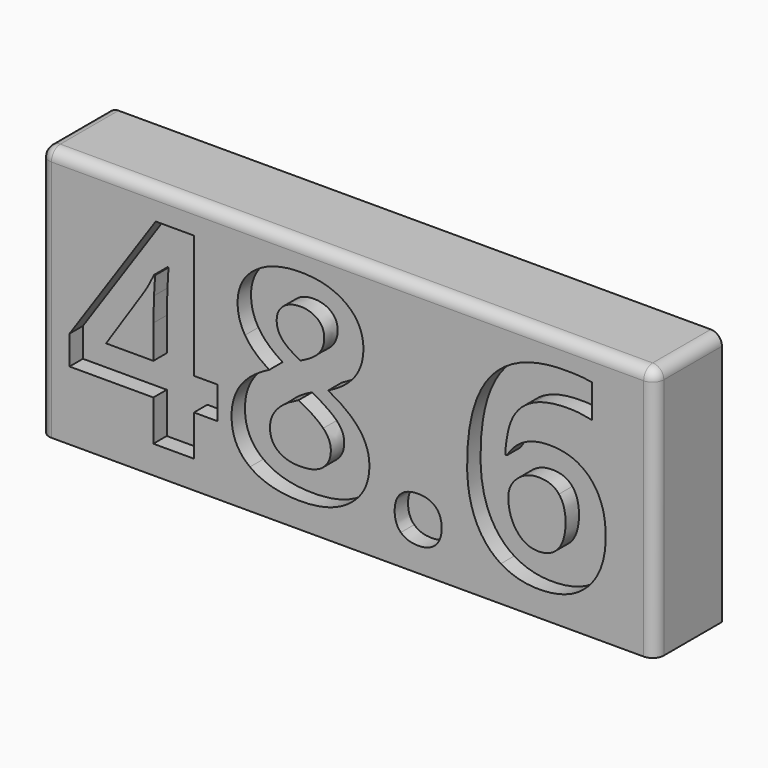
from build123d import *

# Parameters (mm, degrees)
F0_W         = 110
F0_H         = 45.4570637119
F1_DEPTH     = 15
F0_TEXT_SIZE = 49.2459218221
F2_DEPTH     = 12
F3_R         = 2


# Not quite as in the source:
# - Text() gives the source's letters only with a copy of the font that has no kerning and outlines rounded to 1/6400 em; it was checked with that copy


with BuildPart() as f1:
    # F0 (on Front) → F1 (new body)
    with BuildSketch(Plane.XZ):
        with Locations((0.6027820706, 5.2631582404)):
            Rectangle(F0_W, F0_H)
        Polygon((-22.6608187135, 0.5924903425), (-22.6608187135, -5.178516121), (-26.89289012, -5.178516121), (-26.89289012, -12.4653736156), (-34.1566635888, -12.4653736156), (-34.1566635888, -5.178516121), (-49.161280394, -5.178516121), (-49.161280394, -0.0076943297), (-33.7411511234, 22.6915977602), (-26.89289012, 22.6915977602), (-26.89289012, 0.5924903425), align=None, mode=Mode.SUBTRACT)
        with BuildLine():
            add(Edge.make_bspline(
                [(-15.9510618652, 20.8140969907), (-12.8270236996, 23.145583602), (-7.8024007387, 23.145583602)],
                knots=[0, 0, 0, 1, 1, 1], degree=2))
            add(Edge.make_bspline(
                [(-7.8024007387, 23.145583602), (-2.7469990766, 23.145583602), (0.3424130502, 20.8487230295)],
                knots=[0, 0, 0, 1, 1, 1], degree=2))
            add(Edge.make_bspline(
                [(0.3424130502, 20.8487230295), (3.431825177, 18.551862457), (3.431825177, 14.658356763)],
                knots=[0, 0, 0, 1, 1, 1], degree=2))
            add(Edge.make_bspline(
                [(3.431825177, 14.658356763), (3.431825177, 11.9652204133), (1.9390581717, 9.860726723)],
                knots=[0, 0, 0, 1, 1, 1], degree=2))
            add(Edge.make_bspline(
                [(1.9390581717, 9.860726723), (0.4462911665, 7.7562330326), (-2.8701138812, 6.1018778464)],
                knots=[0, 0, 0, 1, 1, 1], degree=2))
            add(Edge.make_bspline(
                [(-2.8701138812, 6.1018778464), (1.0695598646, 3.9858421431), (2.7893197907, 1.6889815706)],
                knots=[0, 0, 0, 1, 1, 1], degree=2))
            add(Edge.make_bspline(
                [(2.7893197907, 1.6889815706), (4.5090797168, -0.6078790019), (4.5090797168, -3.3548780785)],
                knots=[0, 0, 0, 1, 1, 1], degree=2))
            add(Edge.make_bspline(
                [(4.5090797168, -3.3548780785), (4.5090797168, -7.6792855885), (1.1195752539, -10.3147118735)],
                knots=[0, 0, 0, 1, 1, 1], degree=2))
            add(Edge.make_bspline(
                [(1.1195752539, -10.3147118735), (-2.269929209, -12.9501381585), (-7.8024007387, -12.9501381585)],
                knots=[0, 0, 0, 1, 1, 1], degree=2))
            add(Edge.make_bspline(
                [(-7.8024007387, -12.9501381585), (-13.5734072022, -12.9501381585), (-16.8667282241, -10.4955367427)],
                knots=[0, 0, 0, 1, 1, 1], degree=2))
            add(Edge.make_bspline(
                [(-16.8667282241, -10.4955367427), (-20.1600492459, -8.0409353269), (-20.1600492459, -3.5472449606)],
                knots=[0, 0, 0, 1, 1, 1], degree=2))
            add(Edge.make_bspline(
                [(-20.1600492459, -3.5472449606), (-20.1600492459, -0.5386269243), (-18.5595567867, 1.792859687)],
                knots=[0, 0, 0, 1, 1, 1], degree=2))
            add(Edge.make_bspline(
                [(-18.5595567867, 1.792859687), (-16.9590643275, 4.1243462982), (-13.4272083718, 5.9095109643)],
                knots=[0, 0, 0, 1, 1, 1], degree=2))
            add(Edge.make_bspline(
                [(-13.4272083718, 5.9095109643), (-16.4358264081, 7.8024010843), (-17.7554632195, 9.9684521769)],
                knots=[0, 0, 0, 1, 1, 1], degree=2))
            add(Edge.make_bspline(
                [(-17.7554632195, 9.9684521769), (-19.0751000308, 12.1345032696), (-19.0751000308, 14.7045248147)],
                knots=[0, 0, 0, 1, 1, 1], degree=2))
            add(Edge.make_bspline(
                [(-19.0751000308, 14.7045248147), (-19.0751000308, 18.4826103795), (-15.9510618652, 20.8140969907)],
                knots=[0, 0, 0, 1, 1, 1], degree=2))
        make_face(mode=Mode.SUBTRACT)
        with BuildLine():
            add(Edge.make_bspline(
                [(10.1377346876, -12.0421664749), (9.0335487842, -10.9726066104), (9.0335487842, -9.0258537633)],
                knots=[0, 0, 0, 1, 1, 1], degree=2))
            add(Edge.make_bspline(
                [(9.0335487842, -9.0258537633), (9.0335487842, -7.0098488387), (10.1146506617, -5.974915013)],
                knots=[0, 0, 0, 1, 1, 1], degree=2))
            add(Edge.make_bspline(
                [(10.1146506617, -5.974915013), (11.1957525392, -4.9399811872), (13.2656201908, -4.9399811872)],
                knots=[0, 0, 0, 1, 1, 1], degree=2))
            add(Edge.make_bspline(
                [(13.2656201908, -4.9399811872), (15.2585410896, -4.9399811872), (16.35118498, -5.9979990388)],
                knots=[0, 0, 0, 1, 1, 1], degree=2))
            add(Edge.make_bspline(
                [(16.35118498, -5.9979990388), (17.4438288704, -7.0560168905), (17.4438288704, -9.0258537633)],
                knots=[0, 0, 0, 1, 1, 1], degree=2))
            add(Edge.make_bspline(
                [(17.4438288704, -9.0258537633), (17.4438288704, -10.9264385587), (16.3396429671, -12.0190824491)],
                knots=[0, 0, 0, 1, 1, 1], degree=2))
            add(Edge.make_bspline(
                [(16.3396429671, -12.0190824491), (15.2354570637, -13.1117263395), (13.2656201908, -13.1117263395)],
                knots=[0, 0, 0, 1, 1, 1], degree=2))
            add(Edge.make_bspline(
                [(13.2656201908, -13.1117263395), (11.241920591, -13.1117263395), (10.1377346876, -12.0421664749)],
                knots=[0, 0, 0, 1, 1, 1], degree=2))
        make_face(mode=Mode.SUBTRACT)
        with BuildLine():
            add(Edge.make_bspline(
                [(23.5649430594, -5.8787315719), (21.9913819637, -2.4161276938), (21.9913819637, 2.469991112)],
                knots=[0, 0, 0, 1, 1, 1], degree=2))
            add(Edge.make_bspline(
                [(21.9913819637, 2.469991112), (21.9913819637, 12.9039707981), (26.4042782395, 18.0016931742)],
                knots=[0, 0, 0, 1, 1, 1], degree=2))
            add(Edge.make_bspline(
                [(26.4042782395, 18.0016931742), (30.8171745152, 23.0994155503), (39.6198830409, 23.0994155503)],
                knots=[0, 0, 0, 1, 1, 1], degree=2))
            add(Edge.make_bspline(
                [(39.6198830409, 23.0994155503), (42.620806402, 23.0994155503), (44.3290243152, 22.7377658119)],
                knots=[0, 0, 0, 1, 1, 1], degree=2))
            Line((44.3290243152, 22.7377658119), (44.3290243152, 16.7974764921))
            add(Edge.make_bspline(
                [(44.3290243152, 16.7974764921), (42.189904586, 17.2822410351), (40.0969529086, 17.2822410351)],
                knots=[0, 0, 0, 1, 1, 1], degree=2))
            add(Edge.make_bspline(
                [(40.0969529086, 17.2822410351), (36.2726992921, 17.2822410351), (33.8565712527, 16.1280397424)],
                knots=[0, 0, 0, 1, 1, 1], degree=2))
            add(Edge.make_bspline(
                [(33.8565712527, 16.1280397424), (31.4404432133, 14.9738384496), (30.2400738689, 12.7116039159)],
                knots=[0, 0, 0, 1, 1, 1], degree=2))
            add(Edge.make_bspline(
                [(30.2400738689, 12.7116039159), (29.0397045245, 10.4493693822), (28.8242536165, 6.2942447285)],
                knots=[0, 0, 0, 1, 1, 1], degree=2))
            Line((28.8242536165, 6.2942447285), (29.1320406279, 6.2942447285))
            add(Edge.make_bspline(
                [(29.1320406279, 6.2942447285), (31.5173899661, 10.3801173047), (36.757463835, 10.3801173047)],
                knots=[0, 0, 0, 1, 1, 1], degree=2))
            add(Edge.make_bspline(
                [(36.757463835, 10.3801173047), (41.4666051093, 10.3801173047), (44.1366574331, 7.4215146577)],
                knots=[0, 0, 0, 1, 1, 1], degree=2))
            add(Edge.make_bspline(
                [(44.1366574331, 7.4215146577), (46.8067097568, 4.4629120107), (46.8067097568, -0.7540778323)],
                knots=[0, 0, 0, 1, 1, 1], degree=2))
            add(Edge.make_bspline(
                [(46.8067097568, -0.7540778323), (46.8067097568, -6.3788854654), (43.6326562019, -9.664511812)],
                knots=[0, 0, 0, 1, 1, 1], degree=2))
            add(Edge.make_bspline(
                [(43.6326562019, -9.664511812), (40.458602647, -12.9501381585), (34.8337950139, -12.9501381585)],
                knots=[0, 0, 0, 1, 1, 1], degree=2))
            add(Edge.make_bspline(
                [(34.8337950139, -12.9501381585), (30.9402893198, -12.9501381585), (28.0393967375, -11.1457368043)],
                knots=[0, 0, 0, 1, 1, 1], degree=2))
            add(Edge.make_bspline(
                [(28.0393967375, -11.1457368043), (25.1385041551, -9.34133545), (23.5649430594, -5.8787315719)],
                knots=[0, 0, 0, 1, 1, 1], degree=2))
        make_face(mode=Mode.SUBTRACT)
    extrude(amount=F1_DEPTH)



with BuildPart() as f1b:
    # F0 (on Front) → F1, piece 2 (new body)
    with BuildSketch(Plane.XZ):
        with BuildLine():
            add(Edge.make_bspline(
                [(-4.7706986765, 16.7513084404), (-5.9710680209, 17.713142851), (-7.8485687904, 17.713142851)],
                knots=[0, 0, 0, 1, 1, 1], degree=2))
            add(Edge.make_bspline(
                [(-7.8485687904, 17.713142851), (-9.7491535857, 17.713142851), (-10.9148968914, 16.7397664275)],
                knots=[0, 0, 0, 1, 1, 1], degree=2))
            add(Edge.make_bspline(
                [(-10.9148968914, 16.7397664275), (-12.080640197, 15.766390004), (-12.080640197, 14.1274241683)],
                knots=[0, 0, 0, 1, 1, 1], degree=2))
            add(Edge.make_bspline(
                [(-12.080640197, 14.1274241683), (-12.080640197, 12.6885198901), (-11.1534318252, 11.5458606103)],
                knots=[0, 0, 0, 1, 1, 1], degree=2))
            add(Edge.make_bspline(
                [(-11.1534318252, 11.5458606103), (-10.2262234534, 10.4032013305), (-7.8024007387, 9.2028319861)],
                knots=[0, 0, 0, 1, 1, 1], degree=2))
            add(Edge.make_bspline(
                [(-7.8024007387, 9.2028319861), (-5.4401354263, 10.3031705518), (-4.5052323792, 11.4573718445)],
                knots=[0, 0, 0, 1, 1, 1], degree=2))
            add(Edge.make_bspline(
                [(-4.5052323792, 11.4573718445), (-3.5703293321, 12.6115731372), (-3.5703293321, 14.1274241683)],
                knots=[0, 0, 0, 1, 1, 1], degree=2))
            add(Edge.make_bspline(
                [(-3.5703293321, 14.1274241683), (-3.5703293321, 15.7894740298), (-4.7706986765, 16.7513084404)],
                knots=[0, 0, 0, 1, 1, 1], degree=2))
        make_face()
    extrude(amount=F1_DEPTH)


with BuildPart() as f1c:
    # F0 (on Front) → F1, piece 3 (new body)
    with BuildSketch(Plane.XZ):
        with BuildLine():
            add(Edge.make_bspline(
                [(-8.1640504771, 2.8547248762), (-13.2810095414, 0.4924595638), (-13.2810095414, -3.1086484694)],
                knots=[0, 0, 0, 1, 1, 1], degree=2))
            add(Edge.make_bspline(
                [(-13.2810095414, -3.1086484694), (-13.2810095414, -5.178516121), (-11.8382579255, -6.3327174137)],
                knots=[0, 0, 0, 1, 1, 1], degree=2))
            add(Edge.make_bspline(
                [(-11.8382579255, -6.3327174137), (-10.3955063096, -7.4869187064), (-7.8947368421, -7.4869187064)],
                knots=[0, 0, 0, 1, 1, 1], degree=2))
            add(Edge.make_bspline(
                [(-7.8947368421, -7.4869187064), (-5.1323484149, -7.4869187064), (-3.7626962142, -6.2980913749)],
                knots=[0, 0, 0, 1, 1, 1], degree=2))
            add(Edge.make_bspline(
                [(-3.7626962142, -6.2980913749), (-2.3930440135, -5.1092640434), (-2.3930440135, -3.1625111964)],
                knots=[0, 0, 0, 1, 1, 1], degree=2))
            add(Edge.make_bspline(
                [(-2.3930440135, -3.1625111964), (-2.3930440135, -1.5466293866), (-3.7511542013, -0.1423511472)],
                knots=[0, 0, 0, 1, 1, 1], degree=2))
            add(Edge.make_bspline(
                [(-3.7511542013, -0.1423511472), (-5.109264389, 1.2619270923), (-8.1640504771, 2.8547248762)],
                knots=[0, 0, 0, 1, 1, 1], degree=2))
        make_face()
    extrude(amount=F1_DEPTH)


with BuildPart() as f1d:
    # F0 (on Front) → F1, piece 4 (new body)
    with BuildSketch(Plane.XZ):
        with BuildLine():
            Line((-42.620806402, 0.5924903425), (-34.1566635888, 0.5924903425))
            Line((-34.1566635888, 0.5924903425), (-34.1566635888, 6.5558636882))
            add(Edge.make_bspline(
                [(-34.1566635888, 6.5558636882), (-34.1566635888, 8.0486306934), (-34.0335487842, 10.8841185358)],
                knots=[0, 0, 0, 1, 1, 1], degree=2))
            add(Edge.make_bspline(
                [(-34.0335487842, 10.8841185358), (-33.9104339797, 13.7196063782), (-33.8411819021, 14.1812868953)],
                knots=[0, 0, 0, 1, 1, 1], degree=2))
            Line((-33.8411819021, 14.1812868953), (-34.0335487842, 14.1812868953))
            add(Edge.make_bspline(
                [(-34.0335487842, 14.1812868953), (-34.9261311173, 12.2037553472), (-36.1726685134, 10.333949253)],
                knots=[0, 0, 0, 1, 1, 1], degree=2))
            Line((-36.1726685134, 10.333949253), (-42.620806402, 0.5924903425))
        make_face()
    extrude(amount=F1_DEPTH)


with BuildPart() as f1e:
    # F0 (on Front) → F1, piece 5 (new body)
    with BuildSketch(Plane.XZ):
        with BuildLine():
            add(Edge.make_bspline(
                [(30.8748845799, -5.0361646282), (32.379193598, -7.0098488387), (34.6875961834, -7.0098488387)],
                knots=[0, 0, 0, 1, 1, 1], degree=2))
            add(Edge.make_bspline(
                [(34.6875961834, -7.0098488387), (37.0652508464, -7.0098488387), (38.3425669437, -5.4093563795)],
                knots=[0, 0, 0, 1, 1, 1], degree=2))
            add(Edge.make_bspline(
                [(38.3425669437, -5.4093563795), (39.6198830409, -3.8088639203), (39.6198830409, -0.854108611)],
                knots=[0, 0, 0, 1, 1, 1], degree=2))
            add(Edge.make_bspline(
                [(39.6198830409, -0.854108611), (39.6198830409, 1.7236076094), (38.4272083718, 3.2009852641)],
                knots=[0, 0, 0, 1, 1, 1], degree=2))
            add(Edge.make_bspline(
                [(38.4272083718, 3.2009852641), (37.2345337027, 4.6783629187), (34.8337950139, 4.6783629187)],
                knots=[0, 0, 0, 1, 1, 1], degree=2))
            add(Edge.make_bspline(
                [(34.8337950139, 4.6783629187), (32.5715604801, 4.6783629187), (30.9710680209, 3.212527277)],
                knots=[0, 0, 0, 1, 1, 1], degree=2))
            add(Edge.make_bspline(
                [(30.9710680209, 3.212527277), (29.3705755617, 1.7466916352), (29.3705755617, -0.2000612118)],
                knots=[0, 0, 0, 1, 1, 1], degree=2))
            add(Edge.make_bspline(
                [(29.3705755617, -0.2000612118), (29.3705755617, -3.0624804177), (30.8748845799, -5.0361646282)],
                knots=[0, 0, 0, 1, 1, 1], degree=2))
        make_face()
    extrude(amount=F1_DEPTH)


with BuildPart() as f1_1:
    add(f1.part)

    add(f1b.part)  # F2 merges F1b

    add(f1c.part)  # F2 merges F1c

    add(f1d.part)  # F2 merges F1d

    add(f1e.part)  # F2 merges F1e
    # F0 (on Front) → F2 (join)
    with BuildSketch(Plane.XZ):
        with Locations((-50, -12.4653736156)):
            Text('48.6', F0_TEXT_SIZE, font='Open Sans', font_style=FontStyle.BOLD, text_align=(TextAlign.LEFT, TextAlign.BOTTOM))
    extrude(amount=F2_DEPTH)

    # F3
    f3_edges = [f1_1.edges().sort_by_distance(p)[0] for p in [
        (0.602782, -15, 27.99169),
        (-54.397218, -7.5, 27.99169),
        (-54.397218, -15, 5.263158),
        (55.602782, -15, 5.263158),
        (55.602782, -7.5, 27.99169),
    ]]
    fillet(f3_edges, radius=F3_R)


solid = f1_1.part
